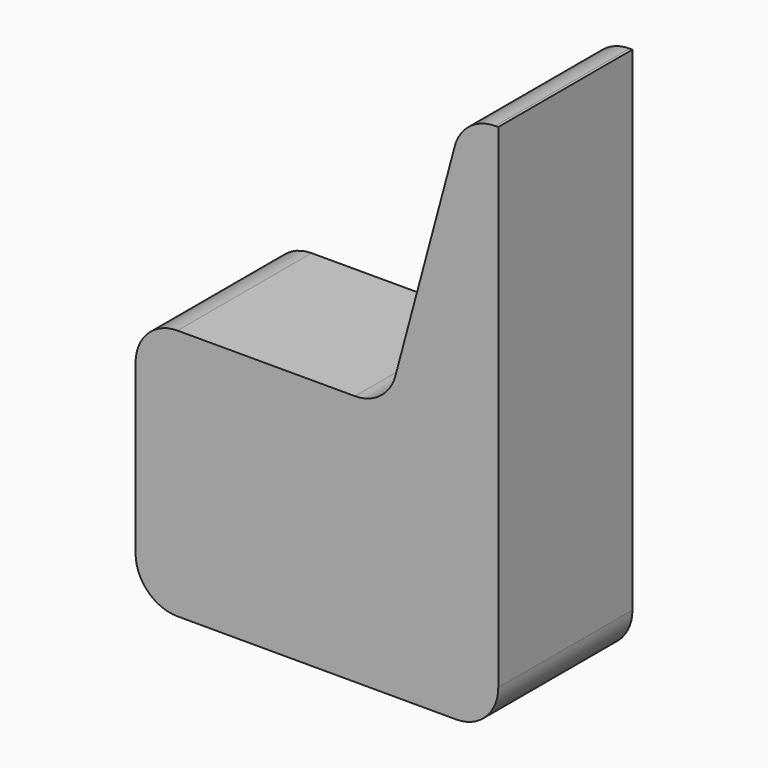
from build123d import *

# Parameters (mm, degrees)
F2_DEPTH = 400
F3_R     = 100


# Not quite as in the source:
# - a feature of the source that left no trace in its solid (it failed there, or was rolled back) is left out
# - the program builds the solid bodies; features that only make, move or delete a surface that nothing else refers to are left out


with BuildPart() as f2:
    # F1 (on offset) → F2 (new body)
    with BuildSketch(Plane.XZ.offset(500)):
        Polygon((-781.1733315718, 197.8861267962), (-781.1733315718, -402.1138732038), (83.9892935576, -402.5302380195), (83.9892935576, 874.0342051986), (0, 874.0342051986), (-181.1733315718, 197.8861267962), align=None)
    extrude(amount=F2_DEPTH)

    # F3
    f3_edges = [f2.edges().sort_by_distance(p)[0] for p in [
        (-781.173332, -700, 197.886127),
        (0, -700, 874.034205),
        (-181.173332, -700, 197.886127),
        (-781.173332, -700, -402.113873),
        (83.989294, -700, -402.530238),
    ]]
    fillet(f3_edges, radius=F3_R)


solid = f2.part
